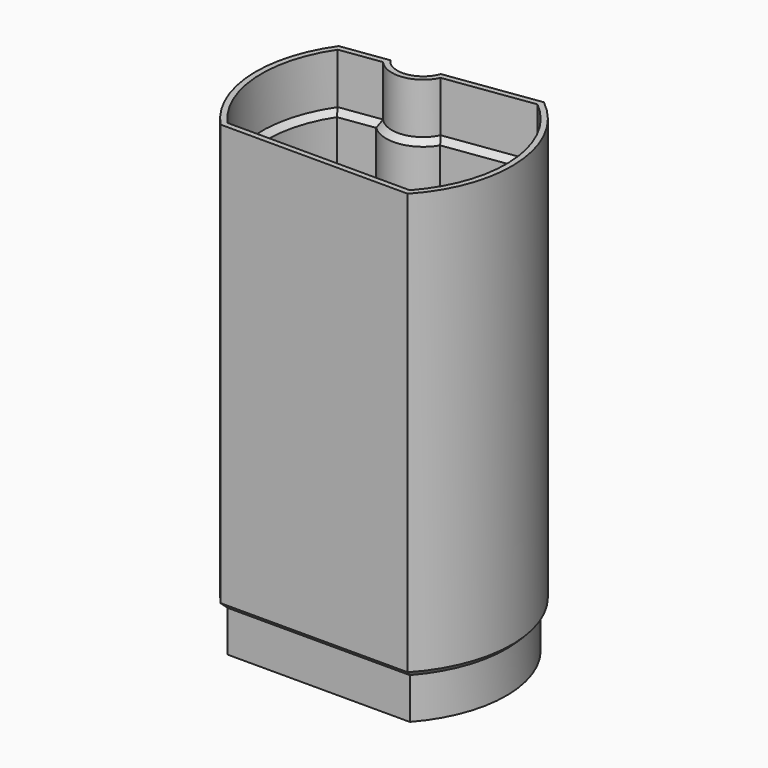
from build123d import *

# Parameters (mm, degrees)
F1_DEPTH = 100
F3_DEPTH = 10
F5_DEPTH = 12
F6_SIZE  = 1.19999


# Not quite as in the source:
# - a fillet or chamfer is up to 0.001 mm smaller than in the source, because OpenCascade refuses the exact size


with BuildPart() as f1:
    # F0 (on Top) → F1 (new body)
    with BuildSketch(Plane.XY):
        with BuildLine():
            Line((-12.0897765349, -15.731314094), (27.9102234651, -15.731314094))
            ThreePointArc((27.9102234651, -15.731314094), (35.186552736, 4.9027765722), (25.0045970812, 24.268685906))
            Line((25.0045970812, 24.268685906), (5.1992357064, 21.4852238868))
            ThreePointArc((5.1992357064, 21.4852238868), (0.7654520553, 17.832613514), (-4.5033702016, 20.1216115537))
            Line((-4.5033702016, 20.1216115537), (-14.406050889, 18.7298805441))
            ThreePointArc((-14.406050889, 18.7298805441), (-19.3764079278, 1.0873626828), (-12.0897765349, -15.731314094))
        make_face()
        with BuildLine():
            ThreePointArc((-11.0175789214, -13.331314094), (-16.9820661814, 1.2521155975), (-13.0181733872, 16.5013478326))
            Line((-13.0181733872, 16.5013478326), (-5.4545185869, 17.5643501916))
            ThreePointArc((-5.4545185869, 17.5643501916), (1.0994674976, 15.455970149), (6.8184149763, 19.2891985189))
            Line((6.8184149763, 19.2891985189), (24.284750464, 21.7439318875))
            ThreePointArc((24.284750464, 21.7439318875), (32.7925833849, 4.7326981573), (26.8380258517, -13.331314094))
            Line((26.8380258517, -13.331314094), (-11.0175789214, -13.331314094))
        make_face(mode=Mode.SUBTRACT)
    extrude(amount=F1_DEPTH)

    # F2 (on face) → F3 (cut)
    with BuildSketch(Plane(origin=(0, 0, 0), x_dir=(1, 0, 0), z_dir=(0, 0, -1))):
        with BuildLine():
            Line((27.9102234651, 15.731314094), (-12.0897765349, 15.731314094))
            ThreePointArc((-12.0897765349, 15.731314094), (-19.3764079278, -1.0873626828), (-14.406050889, -18.7298805441))
            Line((-14.406050889, -18.7298805441), (-4.5033702016, -20.1216115537))
            ThreePointArc((-4.5033702016, -20.1216115537), (0.7654520553, -17.832613514), (5.1992357064, -21.4852238868))
            Line((5.1992357064, -21.4852238868), (25.0045970812, -24.268685906))
            ThreePointArc((25.0045970812, -24.268685906), (35.186552736, -4.9027765722), (27.9102234651, 15.731314094))
        make_face()
        with BuildLine():
            ThreePointArc((6.0462768814, -20.3924746735), (0.9324597764, -16.6442918315), (-5.0163959343, -18.837717402))
            Line((-5.0163959343, -18.837717402), (-13.7193495518, -17.6145970362))
            ThreePointArc((-13.7193495518, -17.6145970362), (-18.1792377522, -1.1697483945), (-11.5610592762, 14.531314094))
            Line((-11.5610592762, 14.531314094), (27.3815062065, 14.531314094))
            ThreePointArc((27.3815062065, 14.531314094), (33.9895674633, -4.8177466261), (24.6519111864, -23.0073260489))
            Line((24.6519111864, -23.0073260489), (6.0462768814, -20.3924746735))
        make_face(mode=Mode.SUBTRACT)
    extrude(amount=-F3_DEPTH, mode=Mode.SUBTRACT)

    # F4 (on face) → F5 (cut)
    with BuildSketch(Plane.XY.offset(100)):
        with BuildLine():
            Line((-5.0163959343, 18.837717402), (-13.7193495518, 17.6145970362))
            ThreePointArc((-13.7193495518, 17.6145970362), (-18.1792377522, 1.1697483945), (-11.5610592762, -14.531314094))
            Line((-11.5610592762, -14.531314094), (27.3815062065, -14.531314094))
            ThreePointArc((27.3815062065, -14.531314094), (33.9895674633, 4.8177466261), (24.6519111864, 23.0073260489))
            Line((24.6519111864, 23.0073260489), (6.0462768814, 20.3924746735))
            ThreePointArc((6.0462768814, 20.3924746735), (0.9324597764, 16.6442918315), (-5.0163959343, 18.837717402))
        make_face()
        with BuildLine():
            ThreePointArc((24.284750464, 21.7439318875), (32.7925833849, 4.7326981573), (26.8380258517, -13.331314094))
            Line((26.8380258517, -13.331314094), (-11.0175789214, -13.331314094))
            ThreePointArc((-11.0175789214, -13.331314094), (-16.9820661814, 1.2521155975), (-13.0181733872, 16.5013478326))
            Line((-13.0181733872, 16.5013478326), (-5.4545185869, 17.5643501916))
            ThreePointArc((-5.4545185869, 17.5643501916), (1.0994674976, 15.455970149), (6.8184149763, 19.2891985189))
            Line((6.8184149763, 19.2891985189), (24.284750464, 21.7439318875))
        make_face(mode=Mode.SUBTRACT)
    extrude(amount=-F5_DEPTH, mode=Mode.SUBTRACT)

    # F6 (size 1.2 in the source; OpenCascade refuses exactly that, so slightly less here)
    f6_edges = [f1.edges().sort_by_distance(p)[0] for p in [
        (15.349094, 21.6999, 10),
        (33.989567, 4.817747, 10),
        (0.93246, 16.644292, 10),
        (-9.367873, 18.226157, 10),
        (-18.179238, 1.169748, 10),
        (7.910223, -14.531314, 10),
        (-18.179238, 1.169748, 88),
        (-9.367873, 18.226157, 88),
        (0.93246, 16.644292, 88),
        (15.349094, 21.6999, 88),
        (7.910223, -14.531314, 88),
        (33.989567, 4.817747, 88),
    ]]
    chamfer(f6_edges, length=F6_SIZE)


solid = f1.part
